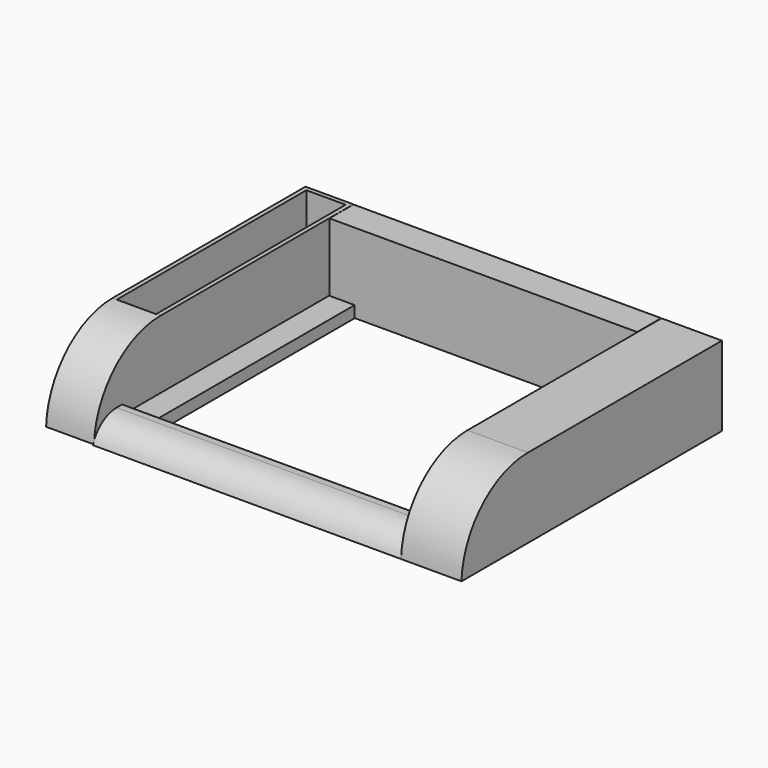
from build123d import *

# Parameters (mm, degrees)
F3_DEPTH       = 46.99
F4_DEPTH       = 6.858
F5_W           = 181.7035898566
F5_H           = 21.5198099613
F6_DEPTH       = 12.446
F7_W           = 28.2824411988
F7_H           = 191.4503723383
F8_DEPTH       = 46.99
F9_W           = 35.6884747744
F9_H           = 192.2272518277
F10_DEPTH      = 46.99
F11_T1_DEPTH   = 273.3487487987
F11_2_T1_DEPTH = 280.7547823743
F12_T1_DEPTH   = 268.7406461084
F13_T          = -2.54


# Not quite as in the source:
# - a fillet or chamfer that OpenCascade refuses, or shapes differently, is made with other operations: its cross-section is extruded or revolved along the edge and cut away or added
# - a shell that OpenCascade refuses in one call is made with other operations: the cavity is built on its own and cut out


with BuildPart() as f3:
    # F2 (on face) → F3 (new body)
    with BuildSketch(Plane.XY):
        Polygon((-90.7814130187, 94.4018736482), (-90.7814130187, 76.682575047), (-76.9056975842, 76.682575047), (77.2037953138, 76.682575047), (90.9062623978, 76.682575047), (90.9062623978, 94.4018736482), align=None)
    extrude(amount=F3_DEPTH)

    # F1 (on face) → F4, piece 2 (join)
    with BuildSketch(Plane.XY):
        Polygon((75.6627693772, 77.2247835994), (75.6627693772, 76.5050277114), (75.7798627019, 76.5050277114), (75.7798627019, -75.7798627019), (75.6627693772, -75.7798627019), (75.6627693772, -78.6267369986), (90.7352864742, -78.6267369986), (90.7352864742, 77.2247835994), align=None)
    extrude(amount=F4_DEPTH)

    # F5 (on face) → F6 (join)
    with BuildSketch(Plane.XY):
        with Locations((0.0419504941, -87.0736762881)):
            Rectangle(F5_W, F5_H)
    extrude(amount=F6_DEPTH)

    # F12: fillet of radius 18.3963073453 on 1 edges, made by hand

    # F12_s2 → F12_t1 (cut)
    with BuildSketch(Plane.YZ.offset(-134.3283725601)):
        with BuildLine():
            ThreePointArc((-80.4261700184, 12.446), (-91.1257130278, 9.0144480263), (-97.8335812688, 0))
            Line((-97.8335812688, 0), (-97.8335812688, 12.446))
            Line((-97.8335812688, 12.446), (-80.4261700184, 12.446))
        make_face()
    extrude(amount=F12_T1_DEPTH, mode=Mode.SUBTRACT)


with BuildPart() as f4:
    # F1 (on face) → F4 (new body)
    with BuildSketch(Plane.XY):
        Polygon((-75.7678225636, 76.5050277114), (-75.7678225636, 76.5324681997), (-90.8200368285, 76.5324681997), (-90.8200368285, -75.8864879608), (-75.7678225636, -75.8864879608), (-75.7678225636, -75.7798627019), (-75.7798701525, -75.7798627019), (-75.7798701525, 76.5050277114), align=None)
    extrude(amount=F4_DEPTH)


with BuildPart() as f8:
    # F7 (on face) → F8 (new body)
    with BuildSketch(Plane.XY):
        with Locations((-105.0322689116, -1.2175962329)):
            Rectangle(F7_W, F7_H)
    extrude(amount=F8_DEPTH)

    # F11: fillet of radius 49.0568195874 on 1 edges, made by hand

    # F11_s2 → F11_t1 (cut)
    with BuildSketch(Plane.YZ.offset(-241.706643311)):
        with BuildLine():
            ThreePointArc((-96.942782402, 0), (-81.8793364369, 33.3447826331), (-47.9295208821, 46.99))
            Line((-47.9295208821, 46.99), (-96.942782402, 46.99))
            Line((-96.942782402, 46.99), (-96.942782402, 0))
        make_face()
    extrude(amount=F11_T1_DEPTH, mode=Mode.SUBTRACT)

    # F13: a shell. OpenCascade refuses it in one call, so the cavity is built on its own and cut out:
    # the body offset inwards by the wall thickness, plus a prism from it out through each open face.
    f13_core = offset(f8.part, amount=F13_T, mode=Mode.PRIVATE)
    f13_exits = [f13_core.faces().sort_by_distance(p)[0] for p in [
        (-105.032269, 22.019035, 44.45),
    ]]
    add(f13_core, mode=Mode.SUBTRACT)
    extrude(f13_exits, amount=-F13_T, mode=Mode.SUBTRACT)


with BuildPart() as f10:
    # F9 (on face) → F10 (new body)
    with BuildSketch(Plane.XY):
        with Locations((108.9476123452, -1.7242766917)):
            Rectangle(F9_W, F9_H)
    extrude(amount=F10_DEPTH)

    # F11#2: fillet of radius 49.0568195874 on 1 edges, made by hand

    # F11_2_s2 → F11_2_t1 (cut)
    with BuildSketch(Plane.YZ.offset(-31.4297788419)):
        with BuildLine():
            ThreePointArc((-97.8379026055, 0), (-82.7744566404, 33.3447826331), (-48.8246410856, 46.99))
            Line((-48.8246410856, 46.99), (-97.8379026055, 46.99))
            Line((-97.8379026055, 46.99), (-97.8379026055, 0))
        make_face()
    extrude(amount=F11_2_T1_DEPTH, mode=Mode.SUBTRACT)


solid = Compound([f3.part, f4.part, f8.part, f10.part])
